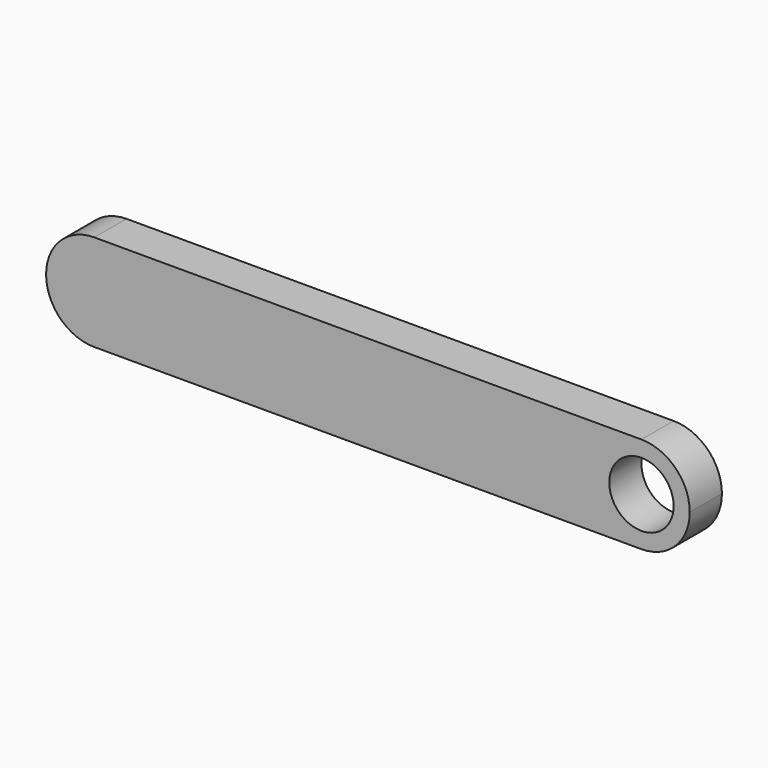
from build123d import *

# Parameters (mm, degrees)
F0_W     = 400
F0_H     = 60
F1_DEPTH = 25
F2_R     = 29.99999
F4_DEPTH = 25


# Not quite as in the source:
# - a fillet or chamfer is up to 0.001 mm smaller than in the source, because OpenCascade refuses the exact size


with BuildPart() as f1:
    # F0 (on Front) → F1 (new body)
    with BuildSketch(Plane.XZ):
        Rectangle(F0_W, F0_H)
    extrude(amount=F1_DEPTH)

    # F2 (radius 30 in the source; OpenCascade refuses exactly that, so slightly less here)
    f2_edges = [f1.edges().sort_by_distance(p)[0] for p in [
        (-200, -12.5, 30),
        (-200, -12.5, -30),
        (200, -12.5, 30),
        (200, -12.5, -30),
    ]]
    fillet(f2_edges, radius=F2_R)

    # F3 (on face) → F4 (cut)
    with BuildSketch(Plane.XZ.offset(25)):
        with BuildLine():
            ThreePointArc((150, 0), (170, -20), (190, 0))
            ThreePointArc((190, 0), (170, 20), (150, 0))
        make_face()
    extrude(amount=-F4_DEPTH, mode=Mode.SUBTRACT)


solid = f1.part
